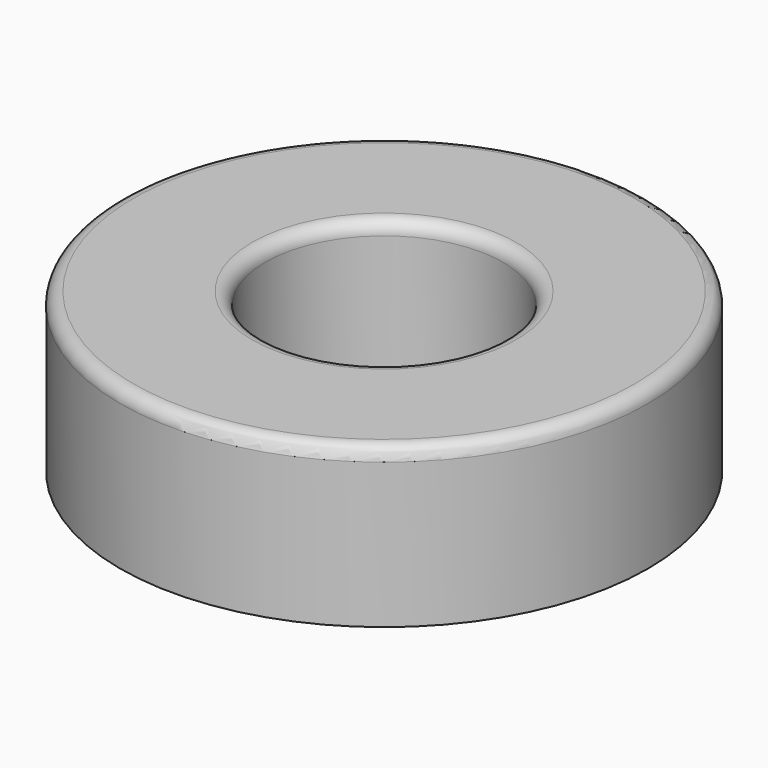
from build123d import *

# Parameters (mm, degrees)
F0_R     = 4
F1_DEPTH = 2.4
F2_D     = 3.6
F3_R     = 0.2


with BuildPart() as f1:
    # F0 (on Top) → F1 (new body)
    with BuildSketch(Plane.XY):
        Circle(F0_R)
    extrude(amount=F1_DEPTH)

    # F2 (through all)
    with Locations(Plane(origin=(0, 0, 0), x_dir=(1, 0, 0), z_dir=(0, 0, -1))):
        with Locations((0, 0)):
            Hole(F2_D / 2)

    # F3
    f3_edges = [f1.edges().sort_by_distance(p)[0] for p in [
        (-4, 0, 2.4),
        (-1.8, 0, 2.4),
    ]]
    fillet(f3_edges, radius=F3_R)


solid = f1.part
